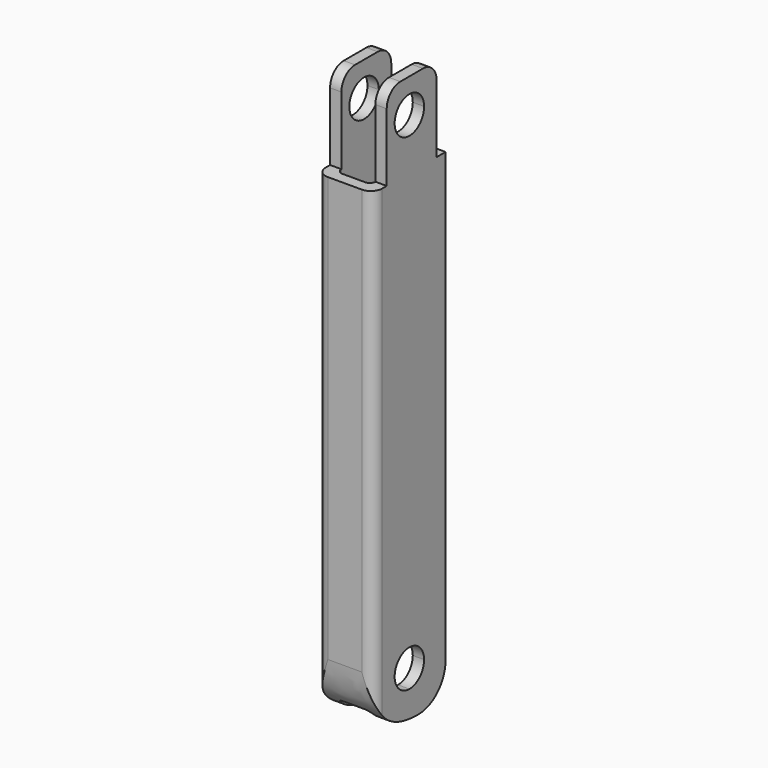
from build123d import *

# Parameters (mm, degrees)
F1_DEPTH    = 100
F2_W        = 2
F2_H        = 15
F2_W_2      = 3
F3_DEPTH    = 25
F4_R        = 3
F5_T1_DEPTH = 56
F6_R        = 5.99999


# Not quite as in the source:
# - a fillet or chamfer that OpenCascade refuses, or shapes differently, is made with other operations: its cross-section is extruded or revolved along the edge and cut away or added
# - a fillet or chamfer is up to 0.001 mm smaller than in the source, because OpenCascade refuses the exact size


with BuildPart() as f1:
    # F0 (on Top) → F1 (new body)
    with BuildSketch(Plane.XY):
        with BuildLine():
            Line((-3.2036672086, -4.7932054844), (-5.2036672086, -4.7932054844))
            Line((-5.2036672086, -4.7932054844), (-5.2036672086, -18.7932054844))
            ThreePointArc((-5.2036672086, -18.7932054844), (-4.6178807709, -20.2074190467), (-3.2036672086, -20.7932054844))
            Line((-3.2036672086, -20.7932054844), (2.7963327914, -20.7932054844))
            ThreePointArc((2.7963327914, -20.7932054844), (4.2105463538, -20.2074190467), (4.7963327914, -18.7932054844))
            Line((4.7963327914, -18.7932054844), (4.7963327914, -4.7932054844))
            Line((4.7963327914, -4.7932054844), (2.7963327914, -4.7932054844))
            Line((2.7963327914, -4.7932054844), (2.7963327914, -17.7932054844))
            ThreePointArc((2.7963327914, -17.7932054844), (2.5034395726, -18.5003122656), (1.7963327914, -18.7932054844))
            Line((1.7963327914, -18.7932054844), (-2.2036672086, -18.7932054844))
            ThreePointArc((-2.2036672086, -18.7932054844), (-2.9107739897, -18.5003122656), (-3.2036672086, -17.7932054844))
            Line((-3.2036672086, -17.7932054844), (-3.2036672086, -4.7932054844))
        make_face()
    extrude(amount=F1_DEPTH)

    # F2 (on face) → F3 (cut)
    with BuildSketch(Plane.YZ.offset(4.7963327914)):
        with BuildLine():
            ThreePointArc((-12.7932054844, 97.25), (-15.0913025232, 91.7019029611), (-9.5432054844, 94))
            ThreePointArc((-9.5432054844, 94), (-10.4951084455, 96.2980970389), (-12.7932054844, 97.25))
        make_face()
        with Locations((-5.7932054844, 92.5)):
            Rectangle(F2_W, F2_H)
        with Locations((-19.2932054844, 92.5)):
            Rectangle(F2_W_2, F2_H)
        with BuildLine():
            ThreePointArc((-12.7932054844, 4.75), (-10.4951084455, 5.7019029611), (-9.5432054844, 8))
            ThreePointArc((-9.5432054844, 8), (-15.0913025232, 10.2980970389), (-12.7932054844, 4.75))
        make_face()
    extrude(amount=-F3_DEPTH, mode=Mode.SUBTRACT)

    # F4
    f4_edges = [f1.edges().sort_by_distance(p)[0] for p in [
        (3.796333, -6.793205, 100),
        (3.796333, -17.793205, 100),
        (-4.203667, -6.793205, 100),
        (-4.203667, -17.793205, 100),
    ]]
    fillet(f4_edges, radius=F4_R)

    # F5: fillet of radius 10 on 1 edges, made by hand

    # F5_s2 → F5_t1 (cut)
    with BuildSketch(Plane.YZ.offset(-28.2036672086)):
        with BuildLine():
            add(Edge.make_bspline(
                [(-10.7932054844, 0), (-20.7932054844, 0), (-20.7932054844, 10)],
                knots=[0, 0, 0, 1, 1, 1], degree=2, weights=[1, 1, 1]))
            Line((-20.7932054844, 10), (-20.9932054844, 10))
            Line((-20.9932054844, 10), (-20.9932054844, -0.2))
            Line((-20.9932054844, -0.2), (-10.7932054844, -0.2))
            Line((-10.7932054844, -0.2), (-10.7932054844, 0))
        make_face()
    extrude(amount=F5_T1_DEPTH, mode=Mode.SUBTRACT)

    # F6 (radius 6 in the source; OpenCascade refuses exactly that, so slightly less here)
    f6_edges = [f1.edges().sort_by_distance(p)[0] for p in [
        (3.796333, -4.793205, 0),
        (-4.203667, -4.793205, 0),
    ]]
    fillet(f6_edges, radius=F6_R)


solid = f1.part
